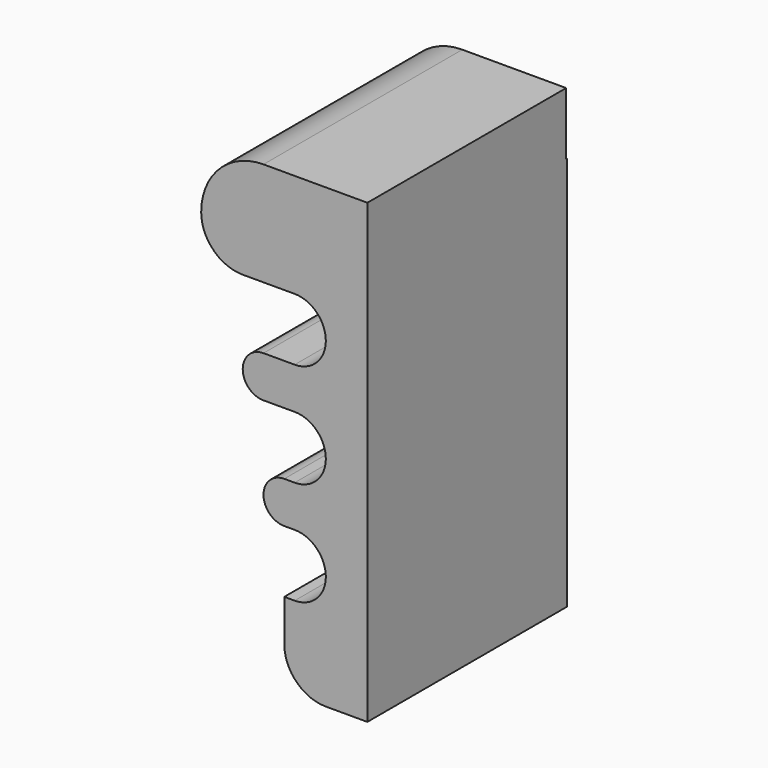
from build123d import *

# Parameters (mm, degrees)
F0_W     = 12.7
F0_H     = 25.4
F0_W_2   = 25.4
F1_DEPTH = 152.4
F2_W     = 152.4
F2_H     = 25.4
F3_DEPTH = 38.1
F4_R     = 25.4
F6_DEPTH = 151.892
F7_R     = 19.05
F8_R     = 19.04999
F9_R     = 19.04999
F10_R    = 12.69999
F11_R    = 25.39999


# Not quite as in the source:
# - a fillet or chamfer is up to 0.001 mm smaller than in the source, because OpenCascade refuses the exact size


with BuildPart() as f1:
    # F0 (on Front) → F1 (new body)
    with BuildSketch(Plane.XZ):
        Polygon((-147.5200289965, 215.9), (-172.9200289965, 215.9), (-249.1200289965, 215.9), (-249.1200289965, 190.5), (-172.9200289965, 190.5), (-172.9200289965, 152.4), (-223.7200289965, 152.4), (-223.7200289965, 127), (-172.9200289965, 127), (-172.9200289965, 88.9), (-211.0200289965, 88.9), (-211.0200289965, 63.5), (-172.9200289965, 63.5), (-172.9200289965, 25.4), (-172.9200289965, 0), (-160.2200289965, 0), (-147.5200289965, 0), (-147.5200289965, 63.5), (-147.5200289965, 88.9), (-147.5200289965, 127), (-147.5200289965, 152.4), (-147.5200289965, 190.5), align=None)
        with Locations((-153.8700289965, -12.7)):
            Rectangle(F0_W, F0_H)
        with Locations((-185.6200289965, 12.7)):
            Rectangle(F0_W_2, F0_H)
    extrude(amount=F1_DEPTH)

    # F2 (on face) → F3 (join)
    with BuildSketch(Plane(origin=(-160.2200289965, 0, 0), x_dir=(0, -1, 0), z_dir=(-1, 0, 0))):
        with Locations((76.2, -12.7)):
            Rectangle(F2_W, F2_H)
    extrude(amount=F3_DEPTH)

    # F4
    f4_edges = [f1.edges().sort_by_distance(p)[0] for p in [
        (-198.320029, -76.2, -25.4),
    ]]
    fillet(f4_edges, radius=F4_R)

    # F5 (on face) → F6 (join)
    with BuildSketch(Plane.XZ.offset(152.4)):
        with BuildLine():
            ThreePointArc((-211.0200289965, 254), (-237.9607973597, 242.8407683632), (-249.1200289965, 215.9))
            Line((-249.1200289965, 215.9), (-147.5200289965, 215.9))
            Line((-147.5200289965, 215.9), (-147.5200289965, 254))
            Line((-147.5200289965, 254), (-211.0200289965, 254))
        make_face()
    extrude(amount=-F6_DEPTH)

    # F7
    f7_edges = [f1.edges().sort_by_distance(p)[0] for p in [
        (-172.920029, -76.2, 88.9),
    ]]
    fillet(f7_edges, radius=F7_R)

    # F8 (radius 19.05 in the source; OpenCascade refuses exactly that, so slightly less here)
    f8_edges = [f1.edges().sort_by_distance(p)[0] for p in [
        (-172.920029, -76.2, 190.5),
        (-172.920029, -76.2, 127),
    ]]
    fillet(f8_edges, radius=F8_R)

    # F9 (radius 19.05 in the source; OpenCascade refuses exactly that, so slightly less here)
    f9_edges = [f1.edges().sort_by_distance(p)[0] for p in [
        (-172.920029, -76.2, 152.4),
        (-172.920029, -76.2, 25.4),
        (-172.920029, -76.2, 63.5),
    ]]
    fillet(f9_edges, radius=F9_R)

    # F10 (radius 12.7 in the source; OpenCascade refuses exactly that, so slightly less here)
    f10_edges = [f1.edges().sort_by_distance(p)[0] for p in [
        (-223.720029, -76.2, 152.4),
        (-223.720029, -76.2, 127),
        (-211.020029, -76.2, 88.9),
        (-211.020029, -76.2, 63.5),
    ]]
    fillet(f10_edges, radius=F10_R)

    # F11 (radius 25.4 in the source; OpenCascade refuses exactly that, so slightly less here)
    f11_edges = [f1.edges().sort_by_distance(p)[0] for p in [
        (-249.120029, -76.2, 190.5),
    ]]
    fillet(f11_edges, radius=F11_R)


solid = f1.part
